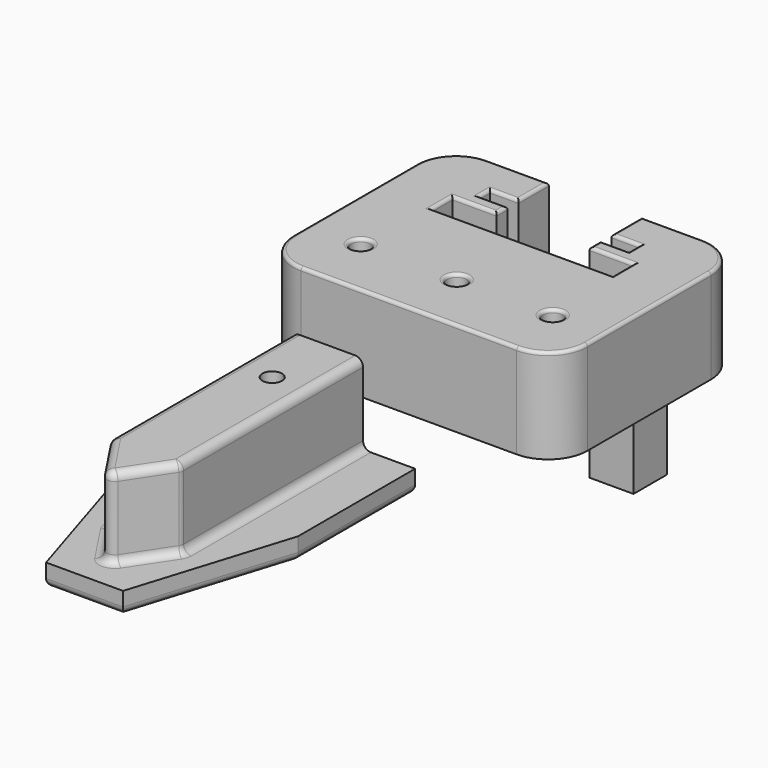
from build123d import *

# Parameters (mm, degrees)
F1_DEPTH      = 3.556
F0_R          = 4.1275
F2_DEPTH      = 16.51
F3_START      = 3.81
F0_R_2        = 1.5875
F3_DEPTH      = 12.7
F4_R          = 1.27
F5_R          = 1.5875
F6_DEPTH      = 15.24
F7_DEPTH      = 15.24
F8_DEPTH      = 17.526
F8_DEPTH_BACK = 15.24
F9_R          = 6.35
F10_R         = 0.508


with BuildPart() as f1:
    # F0 (on Top) → F1 (new body)
    with BuildSketch(Plane.XY):
        Polygon((-5.715, 0), (-14.1224, 0), (-14.1224, -23.622), (-6.20570345, -49.022), (6.20570345, -49.022), (14.1224, -23.622), (14.1224, 0), (5.715, 0), (5.715, -36.576), (0, -45.212), (-5.715, -36.576), align=None)
    extrude(amount=F1_DEPTH)

    # F0 (on Top) → F2 (join)
    with BuildSketch(Plane.XY):
        Polygon((5.715, 0), (-5.715, 0), (-5.715, -36.576), (0, -45.212), (5.715, -36.576), align=None)
        with Locations((0, -11.176)):
            Circle(F0_R, mode=Mode.SUBTRACT)
    extrude(amount=F2_DEPTH)

    # F0 (on Top) → F3 (join)
    with BuildSketch(Plane.XY.offset(F3_START)):
        with Locations((0, -11.176)):
            Circle(F0_R)
        with Locations((0, -11.176)):
            Circle(F0_R_2, mode=Mode.SUBTRACT)
    extrude(amount=F3_DEPTH)

    # F4
    f4_edges = [f1.edges().sort_by_distance(p)[0] for p in [
        (0, -49.022, 0),
        (10.164052, -36.322, 0),
        (14.1224, -11.811, 0),
        (0, 0, 0),
        (-14.1224, -11.811, 0),
        (-10.164052, -36.322, 0),
        (5.715, -18.288, 16.51),
        (-5.715, -18.288, 16.51),
        (-5.715, -36.576, 10.033),
        (5.715, -36.576, 10.033),
        (2.8575, -40.894, 3.556),
        (2.8575, -40.894, 16.51),
        (0, -45.212, 10.033),
        (-2.8575, -40.894, 16.51),
        (5.715, -18.288, 3.556),
        (-2.8575, -40.894, 3.556),
        (-5.715, -18.288, 3.556),
    ]]
    fillet(f4_edges, radius=F4_R)


with BuildPart() as f6:
    # F5 (on Top) → F6 (new body)
    with BuildSketch(Plane.XY):
        Polygon((-23.749, 16.3851472945), (0, 16.3851472945), (23.749, 16.3851472945), (23.749, 53.9771472945), (9.2803988042, 53.9771472945), (9.2803988042, 50.1671472945), (14.605, 50.1671472945), (17.78, 50.1671472945), (17.78, 43.4361472945), (17.78, 36.0701472945), (0, 36.0701472945), (-17.78, 36.0701472945), (-17.78, 43.4361472945), (-17.78, 50.1671472945), (-14.605, 50.1671472945), (-9.2803988042, 50.1671472945), (-9.2803988042, 53.9771472945), (-23.749, 53.9771472945), align=None)
        with Locations((-15.494, 26.0371472945)):
            Circle(F5_R, mode=Mode.SUBTRACT)
        with Locations((0, 26.0371472945)):
            Circle(F5_R, mode=Mode.SUBTRACT)
        with Locations((15.494, 26.0371472945)):
            Circle(F5_R, mode=Mode.SUBTRACT)
    extrude(amount=F6_DEPTH)

    # F5 (on Top) → F7 (join)
    with BuildSketch(Plane.XY):
        Polygon((17.78, 50.1671472945), (14.605, 50.1671472945), (14.605, 43.4361472945), (14.605, 39.2451472945), (0, 39.2451472945), (-14.605, 39.2451472945), (-14.605, 43.4361472945), (-14.605, 50.1671472945), (-17.78, 50.1671472945), (-17.78, 43.4361472945), (-17.78, 36.0701472945), (0, 36.0701472945), (17.78, 36.0701472945), (17.78, 43.4361472945), align=None)
    extrude(amount=F7_DEPTH)

    # F5 (on Top) → F8 (join, two sides)
    with BuildSketch(Plane.XY) as f8_sk:
        Polygon((-7.493, 53.9771472945), (-9.2803988042, 53.9771472945), (-9.2803988042, 50.1671472945), (-14.605, 50.1671472945), (-14.605, 43.4361472945), (-7.493, 43.4361472945), (-7.493, 45.6713472945), (-12.065, 45.6713472945), (-12.065, 47.8811472945), (-7.493, 47.8811472945), align=None)
        Polygon((9.2803988042, 50.1671472945), (9.2803988042, 53.9771472945), (7.493, 53.9771472945), (7.493, 47.8811472945), (12.065, 47.8811472945), (12.065, 45.6713472945), (7.493, 45.6713472945), (7.493, 43.4361472945), (14.605, 43.4361472945), (14.605, 50.1671472945), align=None)
    extrude(amount=-F8_DEPTH)
    extrude(f8_sk.sketch, amount=F8_DEPTH_BACK)

    # F9
    f9_edges = [f6.edges().sort_by_distance(p)[0] for p in [
        (23.749, 53.977147, 7.62),
        (23.749, 16.385147, 7.62),
        (-23.749, 53.977147, 7.62),
        (-23.749, 16.385147, 7.62),
    ]]
    fillet(f9_edges, radius=F9_R)

    # F10
    f10_edges = [f6.edges().sort_by_distance(p)[0] for p in [
        (12.446, 53.977147, 15.24),
        (21.889128, 52.117275, 15.24),
        (23.749, 35.181147, 15.24),
        (21.889128, 18.245019, 15.24),
        (0, 16.385147, 15.24),
        (-21.889128, 18.245019, 15.24),
        (-23.749, 35.181147, 15.24),
        (-21.889128, 52.117275, 15.24),
        (-14.605, 41.340647, 15.24),
        (0, 39.245147, 15.24),
        (14.605, 41.340647, 15.24),
        (11.049, 43.436147, 15.24),
        (-11.049, 43.436147, 15.24),
        (-7.493, 44.553747, 15.24),
        (-12.446, 53.977147, 15.24),
        (7.493, 50.929147, 15.24),
        (-7.493, 50.929147, 15.24),
        (9.779, 47.881147, 15.24),
        (-9.779, 47.881147, 15.24),
        (12.065, 46.776247, 15.24),
        (-12.065, 46.776247, 15.24),
        (9.779, 45.671347, 15.24),
        (-9.779, 45.671347, 15.24),
        (7.493, 44.553747, 15.24),
        (-17.0815, 26.037147, 15.24),
        (-1.5875, 26.037147, 15.24),
        (13.9065, 26.037147, 15.24),
    ]]
    fillet(f10_edges, radius=F10_R)


solid = Compound([f1.part, f6.part])
